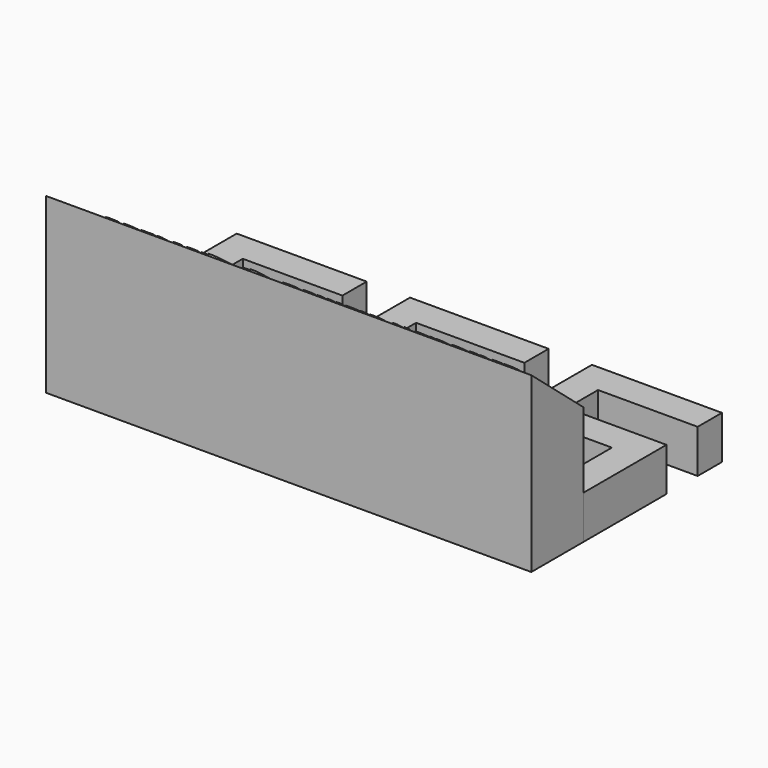
from build123d import *

# Parameters (mm, degrees)
F0_W         = 14.605
F0_H         = 4.445
F0_W_2       = 4.445
F0_W_3       = 10.0838
F0_H_2       = 12.065
F1_DEPTH     = 6.35
F0_W_4       = 15.875
F0_H_3       = 16.51
F0_H_4       = 5.715
F0_W_5       = 10.16
F0_H_5       = 6.35
F2_DEPTH     = 25.4
F4_DEPTH     = 71.121
F5_TEXT_SIZE = 4.5861111111
F6_DEPTH     = 0.635


# Not quite as in the source:
# - Text() gives the source's letters only with a copy of the font that has no kerning and outlines rounded to 1/6400 em; it was checked with that copy


with BuildPart() as f1:
    # F0 (on Top) → F1 (new body)
    with BuildSketch(Plane.XY):
        with Locations((11.7475, 32.7025)):
            Rectangle(F0_W, F0_H)
        with Locations((2.2225, 32.7025)):
            Rectangle(F0_W_2, F0_H)
        with Locations((2.2225, 28.2575)):
            Rectangle(F0_W_2, F0_H)
        with Locations((2.2225, 23.8125)):
            Rectangle(F0_W_2, F0_H)
        with Locations((9.4869, 23.8125)):
            Rectangle(F0_W_3, F0_H)
        with Locations((2.2225, 15.5575)):
            Rectangle(F0_W_2, F0_H_2)
    extrude(amount=F1_DEPTH)


with BuildPart() as f1b:
    # F0 (on Top) → F1, piece 2 (new body)
    with BuildSketch(Plane.XY):
        with Locations((37.7825, 32.7025)):
            Rectangle(F0_W_4, F0_H)
        with Locations((27.6225, 11.7475)):
            Rectangle(F0_W_2, F0_H)
        with Locations((37.7825, 11.7475)):
            Rectangle(F0_W_4, F0_H)
        with Locations((27.6225, 22.225)):
            Rectangle(F0_W_2, F0_H_3)
        with Locations((27.6225, 32.7025)):
            Rectangle(F0_W_2, F0_H)
    extrude(amount=F1_DEPTH)


with BuildPart() as f1c:
    # F0 (on Top) → F1, piece 3 (new body)
    with BuildSketch(Plane.XY):
        with Locations((54.2925, 32.7025)):
            Rectangle(F0_W_2, F0_H)
        with Locations((63.8175, 32.7025)):
            Rectangle(F0_W, F0_H)
        with Locations((54.2925, 27.6225)):
            Rectangle(F0_W_2, F0_H_4)
        with Locations((54.2925, 22.5425)):
            Rectangle(F0_W_2, F0_H)
        with Locations((61.595, 22.5425)):
            Rectangle(F0_W_5, F0_H)
        with Locations((68.8975, 22.5425)):
            Rectangle(F0_W_2, F0_H)
        with Locations((68.8975, 17.145)):
            Rectangle(F0_W_2, F0_H_5)
        with Locations((68.8975, 11.7475)):
            Rectangle(F0_W_2, F0_H)
        with Locations((59.3725, 11.7475)):
            Rectangle(F0_W, F0_H)
    extrude(amount=F1_DEPTH)


with BuildPart() as f2:
    # F0 (on Top) → F2 (new body)
    with BuildSketch(Plane.XY):
        Polygon((0, 9.525), (0, 0), (71.12, 0), (71.12, 9.525), (66.675, 9.525), (52.07, 9.525), (45.72, 9.525), (29.845, 9.525), (25.4, 9.525), (4.445, 9.525), align=None)
    extrude(amount=F2_DEPTH)

    # F3 (on face) → F4 (cut, through all)
    with BuildSketch(Plane.YZ.offset(71.12)):
        Polygon((9.525, 25.4), (0, 25.4), (9.525, 17.407576013), align=None)
    extrude(amount=-F4_DEPTH, mode=Mode.SUBTRACT)

    # F5 (on face) → F6 (join)
    with BuildSketch(Plane(origin=(0, 12.5070584633, 14.9053318564), x_dir=(1, 0, 0), z_dir=(0, 0.6427876097, 0.7660444431))):
        with Locations((4.8506117622, -11.7608030706)):
            Text('Courtesy of Genisis Robotics', F5_TEXT_SIZE, font='Open Sans', font_style=FontStyle.BOLDITALIC, text_align=(TextAlign.LEFT, TextAlign.BOTTOM))
    extrude(amount=F6_DEPTH)


solid = Compound([f1.part, f1b.part, f1c.part, f2.part])
